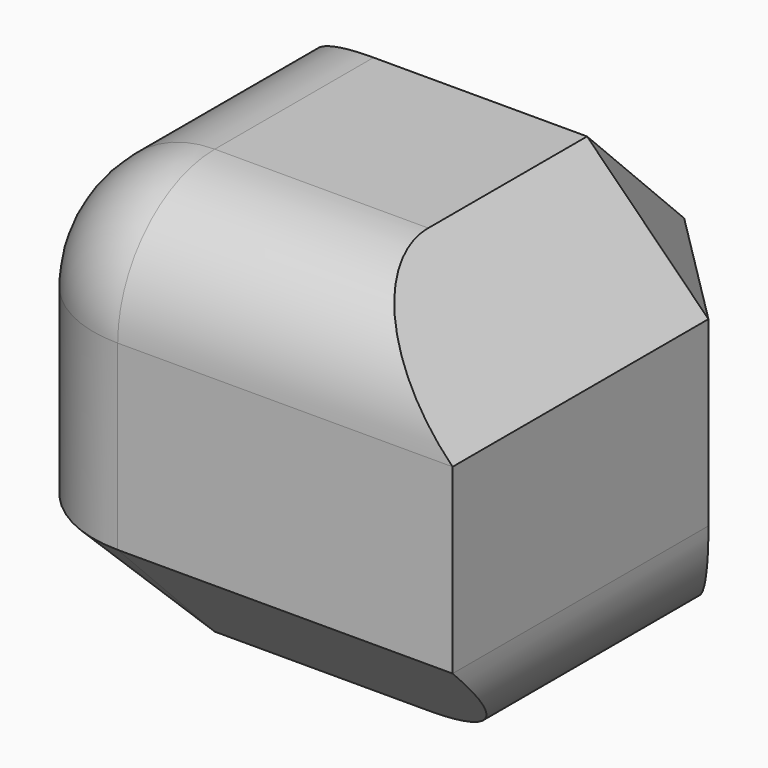
from build123d import *

# Parameters (mm, degrees)
F0_W         = 75.1911774278
F0_H         = 72.7032572031
F1_DEPTH     = 70
F2_R         = 20
F3_T1_DEPTH  = 25.4034118443
F3_T3_DEPTH  = 155.5705767217
F3_T5_DEPTH  = 158.0584969464
F3_T7_DEPTH  = 152.8673195186
F3_T9_DEPTH  = 86.6248371871
F3_T11_DEPTH = 84.1369169624
F3_T14_ANGLE = 90


# Not quite as in the source:
# - a fillet or chamfer that OpenCascade refuses, or shapes differently, is made with other operations: its cross-section is extruded or revolved along the edge and cut away or added


with BuildPart() as f1:
    # F0 (on Top) → F1 (new body)
    with BuildSketch(Plane.XY):
        Rectangle(F0_W, F0_H)
    extrude(amount=F1_DEPTH)

    # F2
    f2_edges = [f1.edges().sort_by_distance(p)[0] for p in [
        (-37.595589, 0, 70),
        (0, -36.351629, 70),
        (-37.595589, -36.351629, 35),
        (0, 36.351629, 0),
        (37.595589, 0, 0),
    ]]
    fillet(f2_edges, radius=F2_R)

    # F3: chamfer of 20 on 6 edges, made by hand

    # F3_s2 → F3_t1 (cut)
    with BuildSketch(Plane(origin=(34.6490724385, 34.6490724385, 34.6490724385), x_dir=(-0.7071067812, 0.7071067812, 0), z_dir=(0.5773502692, 0.5773502692, 0.5773502692))):
        Polygon((-15.0217482547, 18.8009698021), (13.2625229928, 18.8009698021), (-0.879612631, 43.2958672299), align=None)
    extrude(amount=F3_T1_DEPTH, mode=Mode.SUBTRACT)

    # F3_s4 → F3_t3 (cut)
    with BuildSketch(Plane.XZ.offset(-87.7852883609)):
        Polygon((37.5955887139, 50), (17.5955887139, 70), (37.5955887139, 70), align=None)
    extrude(amount=F3_T3_DEPTH, mode=Mode.SUBTRACT)

    # F3_s6 → F3_t5 (cut)
    with BuildSketch(Plane.YZ.offset(-69.0292484732)):
        Polygon((36.3516286016, 50), (16.3516286016, 70), (36.3516286016, 70), align=None)
    extrude(amount=F3_T5_DEPTH, mode=Mode.SUBTRACT)

    # F3_s8 → F3_t7 (cut)
    with BuildSketch(Plane.XY.offset(-31.4336597593)):
        Polygon((37.5955887139, 16.3516286016), (17.5955887139, 36.3516286016), (37.5955887139, 36.3516286016), align=None)
    extrude(amount=F3_T7_DEPTH, mode=Mode.SUBTRACT)

    # F3_s10 → F3_t9 (cut)
    with BuildSketch(Plane.YZ.offset(-17.5955887139)):
        Polygon((-36.3516286016, 20), (-16.3516286016, 0), (-36.3516286016, 0), align=None)
    extrude(amount=F3_T9_DEPTH, mode=Mode.SUBTRACT)

    # F3_s12 → F3_t11 (cut)
    with BuildSketch(Plane.XZ.offset(-67.7852883609)):
        Polygon((-17.5955887139, 0), (-37.5955887139, 20), (-37.5955887139, 0), align=None)
    extrude(amount=F3_T11_DEPTH, mode=Mode.SUBTRACT)

    # F3_s13 → F3_t14 (revolve, cut)
    with BuildSketch(Plane.XZ.offset(16.3516286016)):
        Polygon((-17.5955887139, 0), (-37.5955887139, 20), (-37.5955887139, 0), align=None)
    revolve(axis=Axis((-17.5955887139, -16.3516286016, 0), (0, 0, 1)), revolution_arc=F3_T14_ANGLE, mode=Mode.SUBTRACT)


solid = f1.part
